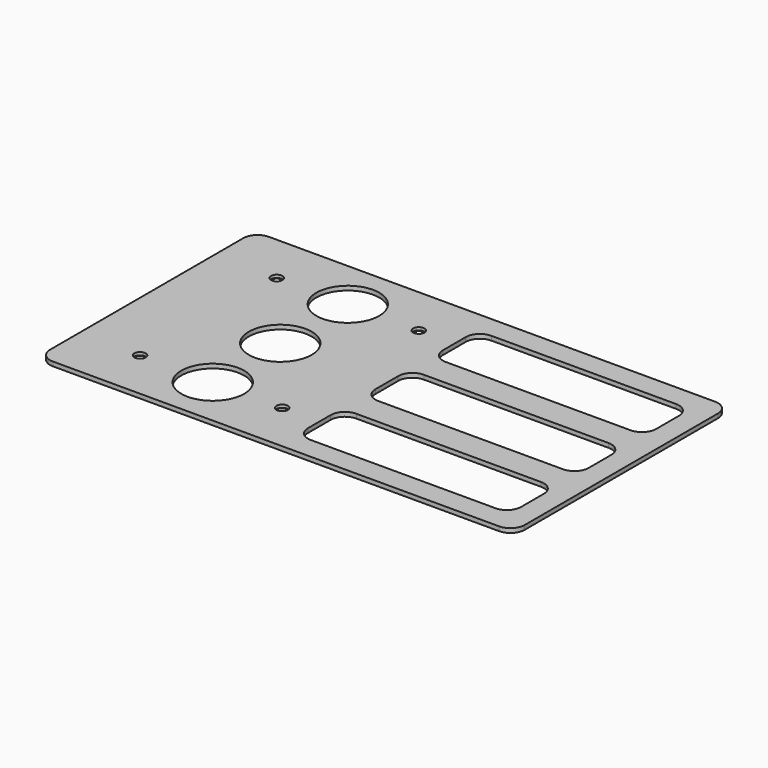
from build123d import *

# Parameters (mm, degrees)
F0_W     = 167
F0_H     = 95
F0_R     = 2
F0_R_2   = 11.05
F0_W_2   = 75
F0_H_2   = 20
F1_DEPTH = 0.75
F2_R     = 5
F3_R     = 5
F4_SIZE  = 0.5


# Not quite as in the source:
# - a feature names something its author has since deleted; it is built from what else it names


with BuildPart() as f1:
    # F0 (on Top) → F1 (new body, symmetric)
    with BuildSketch(Plane.XY):
        with Locations((36.5, 0)):
            Rectangle(F0_W, F0_H)
        with Locations((-25.5706578493, -29.7)):
            Circle(F0_R, mode=Mode.SUBTRACT)
        with Locations((0, -29.7)):
            Circle(F0_R_2, mode=Mode.SUBTRACT)
        with Locations((24.4293421507, -29.7)):
            Circle(F0_R, mode=Mode.SUBTRACT)
        with Locations((75, -29.7)):
            Rectangle(F0_W_2, F0_H_2, mode=Mode.SUBTRACT)
        Circle(F0_R_2, mode=Mode.SUBTRACT)
        with Locations((-25, 29.7)):
            Circle(F0_R, mode=Mode.SUBTRACT)
        with Locations((0, 29.7)):
            Circle(F0_R_2, mode=Mode.SUBTRACT)
        with Locations((25, 29.7)):
            Circle(F0_R, mode=Mode.SUBTRACT)
        with Locations((75, 0)):
            Rectangle(F0_W_2, F0_H_2, mode=Mode.SUBTRACT)
        with Locations((75, 29.7)):
            Rectangle(F0_W_2, F0_H_2, mode=Mode.SUBTRACT)
    extrude(amount=F1_DEPTH, both=True)

    # F2
    f2_edges = [f1.edges().sort_by_distance(p)[0] for p in [
        (120, 47.5, 0),
        (120, -47.5, 0),
        (-47, -47.5, 0),
        (-47, 47.5, 0),
    ]]
    fillet(f2_edges, radius=F2_R)

    # F3
    f3_edges = [f1.edges().sort_by_distance(p)[0] for p in [
        (37.5, 39.7, 0),
        (37.5, 10, 0),
        (37.5, -19.7, 0),
        (112.5, 39.7, 0),
        (112.5, 10, 0),
        (112.5, -19.7, 0),
        (112.5, -39.7, 0),
        (112.5, -10, 0),
        (112.5, 19.7, 0),
        (37.5, -39.7, 0),
        (37.5, -10, 0),
        (37.5, 19.7, 0),
    ]]
    fillet(f3_edges, radius=F3_R)

    # F4
    f4_edges = [f1.edges().sort_by_distance(p)[0] for p in [
        (-27.570658, -29.7, -0.75),
        (22.429342, -29.7, -0.75),
        (23, 29.7, -0.75),
        (-27, 29.7, -0.75),
    ]]
    chamfer(f4_edges, length=F4_SIZE)


solid = f1.part
